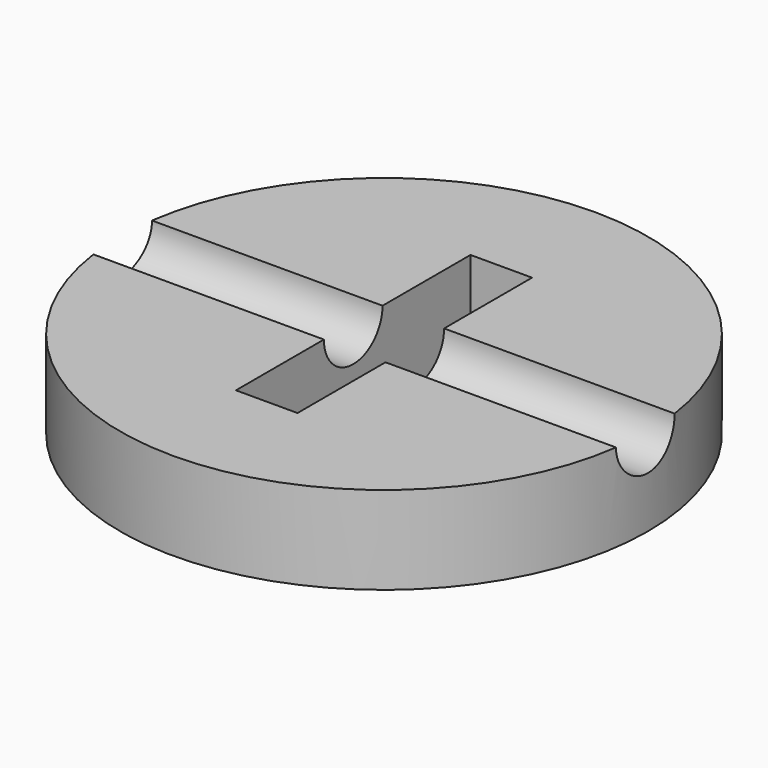
from build123d import *

# Parameters (mm, degrees)
F0_R     = 9
F1_DEPTH = 3
F2_R     = 5.5
F3_DEPTH = 1
F4_R     = 1.25
F5_DEPTH = 9
F6_W     = 2.1
F6_H     = 3.75
F6_H_2   = 2.5
F7_DEPTH = 4.001


# Not quite as in the source:
# - a feature names something its author has since deleted; it is built from what else it names


with BuildPart() as f1:
    # F0 (on Top) → F1 (new body)
    with BuildSketch(Plane.XY):
        Circle(F0_R)
    extrude(amount=-F1_DEPTH)

    # F2 (on face) → F3 (join)
    with BuildSketch(Plane(origin=(0, 0, -3), x_dir=(1, 0, 0), z_dir=(0, 0, -1))):
        Circle(F2_R)
    extrude(amount=F3_DEPTH)

    # F4 (on Right) → F5 (cut, symmetric)
    with BuildSketch(Plane.YZ):
        Circle(F4_R)
    extrude(amount=F5_DEPTH, both=True, mode=Mode.SUBTRACT)

    # F6 (on face) → F7 (cut, through all)
    with BuildSketch(Plane.XY):
        with Locations((0, -3.125)):
            Rectangle(F6_W, F6_H)
        Rectangle(F6_W, F6_H_2)
        with Locations((0, 3.125)):
            Rectangle(F6_W, F6_H)
    extrude(amount=-F7_DEPTH, mode=Mode.SUBTRACT)


solid = f1.part
